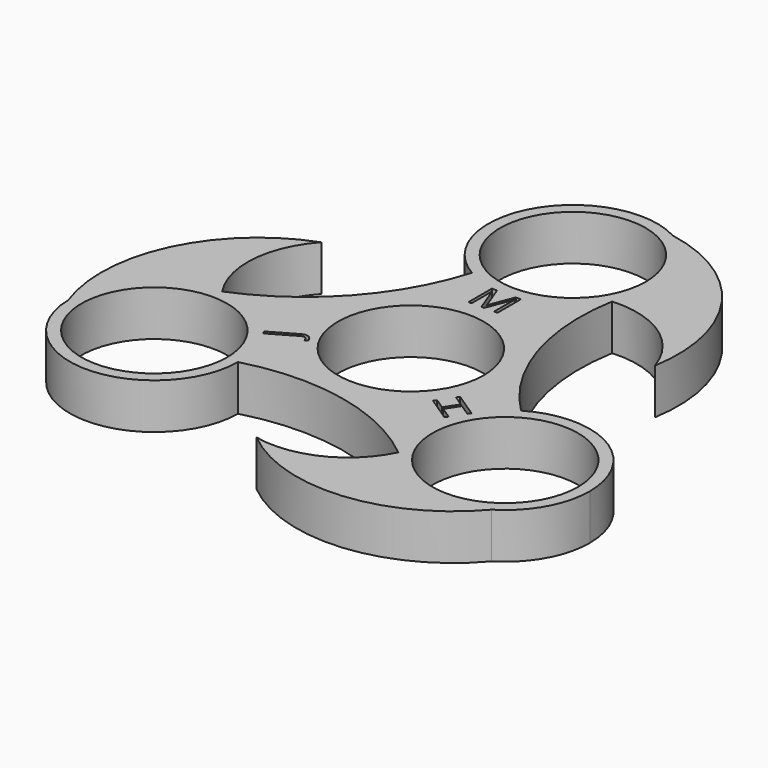
from build123d import *

# Parameters (mm, degrees)
F0_R           = 11.2
F1_DEPTH       = 7
F2_TEXT_SIZE   = 6.3038722274
F2_TEXT_SIZE_2 = 6.2745098039
F3_DEPTH       = 2


# Not quite as in the source:
# - Text() gives the source's letters only with a copy of the font that has no kerning and outlines rounded to 1/6400 em; it was checked with that copy


with BuildPart() as f1:
    # F0 (on Top) → F1 (new body)
    with BuildSketch(Plane.XY):
        with BuildLine():
            ThreePointArc((11.2430318562, 24.6339878555), (12.5530756018, 27.7810213375), (13, 31.1604137288))
            ThreePointArc((13, 31.1604137288), (11.1729239219, 37.8061470244), (6.2052659945, 42.5838402698))
            ThreePointArc((6.2052659945, 42.5838402698), (-11.3219741497, 37.5489113107), (-6.570070942, 19.9428307531))
            ThreePointArc((-6.570070942, 19.9428307531), (3.3107219253, 18.5890526118), (11.2430318562, 24.6339878555))
        make_face()
        with Locations((0, 31.1604137288)):
            Circle(F0_R, mode=Mode.SUBTRACT)
        with BuildLine():
            ThreePointArc((6.2052659945, 42.5838402698), (11.1729239219, 37.8061470244), (13, 31.1604137288))
            ThreePointArc((13, 31.1604137288), (12.5530756018, 27.7810213375), (11.2430318562, 24.6339878555))
            ThreePointArc((11.2430318562, 24.6339878555), (20.164910324, 22.2068441235), (25.6858075207, 14.7899285764))
            ThreePointArc((25.6858075207, 14.7899285764), (21.6625939772, 32.6939263898), (6.2052659945, 42.5838402698))
        make_face()
        with BuildLine():
            ThreePointArc((20.4331293708, -4.3523981445), (12.2966118155, 9.0179765918), (11.2430318562, 24.6339878555))
            ThreePointArc((11.2430318562, 24.6339878555), (3.3107219253, 18.5890526118), (-6.570070942, 19.9428307531))
            ThreePointArc((-6.570070942, 19.9428307531), (-14.1905641992, 6.3592236869), (-26.9448470723, -2.5802710864))
            ThreePointArc((-26.9448470723, -2.5802710864), (-17.7788858765, -6.4022772645), (-13.9857098816, -15.5802068644))
            ThreePointArc((-13.9857098816, -15.5802068644), (-13.9859150141, -15.6532370237), (-13.9865304053, -15.7262648782))
            ThreePointArc((-13.9865304053, -15.7262648782), (1.6239196844, -15.2591587197), (15.6978678096, -22.0288207742))
            ThreePointArc((15.6978678096, -22.0288207742), (14.4284749658, -12.2163026935), (20.4331293708, -4.3523981445))
        make_face()
        Circle(F0_R, mode=Mode.SUBTRACT)
        with BuildLine():
            ThreePointArc((39.9857098816, -15.5802068644), (33.4593662426, -4.3067081475), (20.4331293708, -4.3523981445))
            ThreePointArc((20.4331293708, -4.3523981445), (14.4284749658, -12.2163026935), (15.6978678096, -22.0288207742))
            ThreePointArc((15.6978678096, -22.0288207742), (15.7076014229, -22.0368159701), (15.7173319809, -22.0448148843))
            ThreePointArc((15.7173319809, -22.0448148843), (15.7149535612, -22.0496548048), (15.7125732981, -22.054493819))
            ThreePointArc((15.7125732981, -22.054493819), (23.7673216618, -28.1755225519), (33.7711176275, -26.6688606024))
            ThreePointArc((33.7711176275, -26.6688606024), (38.326130965, -21.9359011342), (39.9857098816, -15.5802068644))
        make_face()
        with Locations((26.9857098816, -15.5802068644)):
            Circle(F0_R, mode=Mode.SUBTRACT)
        with BuildLine():
            ThreePointArc((-13.9857098816, -15.5802068644), (-17.7788858765, -6.4022772645), (-26.9448470723, -2.5802710864))
            ThreePointArc((-26.9448470723, -2.5802710864), (-36.2716671157, -6.4823500703), (-39.9820878811, -15.8870600745))
            ThreePointArc((-39.9820878811, -15.8870600745), (-26.9053000821, -28.5799581799), (-13.9865304053, -15.7262648782))
            ThreePointArc((-13.9865304053, -15.7262648782), (-13.9859150141, -15.6532370237), (-13.9857098816, -15.5802068644))
        make_face()
        with Locations((-26.9857098816, -15.5802068644)):
            Circle(F0_R, mode=Mode.SUBTRACT)
        with BuildLine():
            ThreePointArc((-39.9820878811, -15.8870600745), (-36.2716671157, -6.4823500703), (-26.9448470723, -2.5802710864))
            ThreePointArc((-26.9448470723, -2.5802710864), (-29.3038181756, 6.3598741821), (-25.6410294925, 14.8495691796))
            ThreePointArc((-25.6410294925, 14.8495691796), (-39.1277897708, 2.4282738247), (-39.9820878811, -15.8870600745))
        make_face()
        with BuildLine():
            ThreePointArc((15.7173319809, -22.0448148843), (15.7076014229, -22.0368159701), (15.6978678096, -22.0288207742))
            ThreePointArc((15.6978678096, -22.0288207742), (15.7052132502, -22.0416614801), (15.7125732981, -22.054493819))
            ThreePointArc((15.7125732981, -22.054493819), (15.7149535612, -22.0496548048), (15.7173319809, -22.0448148843))
        make_face()
        with BuildLine():
            ThreePointArc((-0.0292612634, -29.6305958713), (17.4798599433, -35.0990746101), (33.7711176275, -26.6688606024))
            ThreePointArc((33.7711176275, -26.6688606024), (23.7673216618, -28.1755225519), (15.7125732981, -22.054493819))
            ThreePointArc((15.7125732981, -22.054493819), (9.1495657906, -28.5601559768), (-0.0292612634, -29.6305958713))
        make_face()
    extrude(amount=F1_DEPTH)

    # F2 (on face) → F3 (cut)
    with BuildSketch(Plane.XY.offset(7)):
        with Locations((-2.7421844189, 13.7353407228)):
            Text('M', F2_TEXT_SIZE, font='Open Sans', text_align=(TextAlign.LEFT, TextAlign.BOTTOM))
        with Locations(Location((-12.1006091109, -6.2782380965), (0, 0, 120))):
            Text('J', F2_TEXT_SIZE_2, font='Open Sans', text_align=(TextAlign.LEFT, TextAlign.BOTTOM))
        with Locations(Location((13.9883312751, -11.9669613415), (0, 0, 56.3862136283))):
            Text('H', F2_TEXT_SIZE, font='Open Sans', text_align=(TextAlign.LEFT, TextAlign.BOTTOM))
    extrude(amount=-F3_DEPTH, mode=Mode.SUBTRACT)


solid = f1.part
